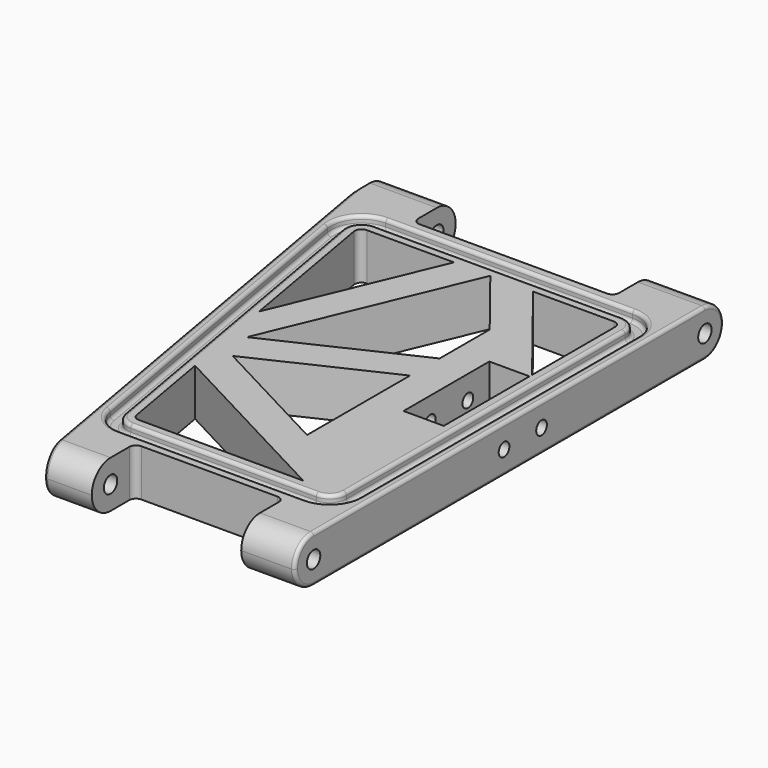
from build123d import *

# Parameters (mm, degrees)
F1_DEPTH  = 3.5
F3_R      = 1.25
F4_DEPTH  = 50.001
F3_R_2    = 1
F5_DEPTH  = 15
F7_DEPTH  = 1.5
F8_R      = 0.5
F9_R      = 0.5
F10_R     = 0.5
F11_R     = 0.5
F13_DEPTH = 1.5
F14_R     = 0.5
F15_R     = 0.5


with BuildPart() as f1:
    # F0 (on Top) → F1 (new body, symmetric)
    with BuildSketch(Plane.XY):
        with BuildLine():
            Line((-29, 45.9712314761), (-39, 45.9712314761))
            Line((-39, 45.9712314761), (-39, 37.9712314761))
            Line((-39, 37.9712314761), (-26.304457389, -34.0287685239))
            Line((-26.304457389, -34.0287685239), (-19.304457389, -34.0287685239))
            Line((-19.304457389, -34.0287685239), (-19.304457389, -27.0287685239))
            ThreePointArc((-19.304457389, -27.0287685239), (-19.0115641702, -26.3216617427), (-18.304457389, -26.0287685239))
            Line((-18.304457389, -26.0287685239), (2, -26.0287685239))
            ThreePointArc((2, -26.0287685239), (2.7071067812, -26.3216617427), (3, -27.0287685239))
            Line((3, -27.0287685239), (3, -34.0287685239))
            Line((3, -34.0287685239), (11, -34.0287685239))
            Line((11, -34.0287685239), (11, 45.9712314761))
            Line((11, 45.9712314761), (1, 45.9712314761))
            Line((1, 45.9712314761), (1, 38.9712314761))
            ThreePointArc((1, 38.9712314761), (0.7071067812, 38.2641246949), (0, 37.9712314761))
            Line((0, 37.9712314761), (-28, 37.9712314761))
            ThreePointArc((-28, 37.9712314761), (-28.7071067812, 38.2641246949), (-29, 38.9712314761))
            Line((-29, 38.9712314761), (-29, 45.9712314761))
        make_face()
        with BuildLine():
            ThreePointArc((5, 36.4712314761), (8.1819805153, 35.1532119914), (9.5, 31.9712314761))
            Line((9.5, 31.9712314761), (9.5, -20.0287685239))
            ThreePointArc((9.5, -20.0287685239), (8.1819805153, -23.2107490392), (5, -24.5287685239))
            Line((5, -24.5287685239), (-22.6804754476, -24.5287685239))
            ThreePointArc((-22.6804754476, -24.5287685239), (-25.5730196912, -23.4759685179), (-27.1121103361, -20.8101853234))
            Line((-27.1121103361, -20.8101853234), (-36.281113333, 31.1898146766))
            ThreePointArc((-36.281113333, 31.1898146766), (-35.2966784385, 34.8637757197), (-31.8494784444, 36.4712314761))
            Line((-31.8494784444, 36.4712314761), (5, 36.4712314761))
        make_face(mode=Mode.SUBTRACT)
        with BuildLine():
            Line((9.5, -20.0287685239), (9.5, 31.9712314761))
            ThreePointArc((9.5, 31.9712314761), (8.1819805153, 35.1532119914), (5, 36.4712314761))
            Line((5, 36.4712314761), (-31.8494784444, 36.4712314761))
            ThreePointArc((-31.8494784444, 36.4712314761), (-35.2966784385, 34.8637757197), (-36.281113333, 31.1898146766))
            Line((-36.281113333, 31.1898146766), (-27.1121103361, -20.8101853234))
            ThreePointArc((-27.1121103361, -20.8101853234), (-25.5730196912, -23.4759685179), (-22.6804754476, -24.5287685239))
            Line((-22.6804754476, -24.5287685239), (5, -24.5287685239))
            ThreePointArc((5, -24.5287685239), (8.1819805153, -23.2107490392), (9.5, -20.0287685239))
        make_face()
        with BuildLine():
            ThreePointArc((5, 34.4712314761), (6.767766953, 33.7389984291), (7.5, 31.9712314761))
            Line((7.5, 31.9712314761), (7.5, -20.0287685239))
            ThreePointArc((7.5, -20.0287685239), (6.767766953, -21.7965354769), (5, -22.5287685239))
            Line((5, -22.5287685239), (-22.6804754476, -22.5287685239))
            ThreePointArc((-22.6804754476, -22.5287685239), (-24.2874444718, -21.9438796317), (-25.1424948301, -20.4628889681))
            Line((-25.1424948301, -20.4628889681), (-34.311497827, 31.5371110319))
            ThreePointArc((-34.311497827, 31.5371110319), (-33.7645895522, 33.5782005003), (-31.8494784444, 34.4712314761))
            Line((-31.8494784444, 34.4712314761), (5, 34.4712314761))
        make_face(mode=Mode.SUBTRACT)
        with BuildLine():
            Line((7.5, -20.0287685239), (7.5, 31.9712314761))
            ThreePointArc((7.5, 31.9712314761), (6.767766953, 33.7389984291), (5, 34.4712314761))
            Line((5, 34.4712314761), (-31.8494784444, 34.4712314761))
            ThreePointArc((-31.8494784444, 34.4712314761), (-33.7645895522, 33.5782005003), (-34.311497827, 31.5371110319))
            Line((-34.311497827, 31.5371110319), (-25.1424948301, -20.4628889681))
            ThreePointArc((-25.1424948301, -20.4628889681), (-24.2874444718, -21.9438796317), (-22.6804754476, -22.5287685239))
            Line((-22.6804754476, -22.5287685239), (5, -22.5287685239))
            ThreePointArc((5, -22.5287685239), (6.767766953, -21.7965354769), (7.5, -20.0287685239))
        make_face()
        with BuildLine():
            Line((6, -17.5660868453), (6, -20.0287685239))
            ThreePointArc((6, -20.0287685239), (5.7071067812, -20.7358753051), (5, -21.0287685239))
            Line((5, -21.0287685239), (1.851729083, -21.0287685239))
            Line((1.851729083, -21.0287685239), (-22.6804754476, -21.0287685239))
            ThreePointArc((-22.6804754476, -21.0287685239), (-23.3232630573, -20.794812967), (-23.6652832006, -20.2024167016))
            Line((-23.6652832006, -20.2024167016), (-26.1277423997, -6.2371166142))
            Line((-26.1277423997, -6.2371166142), (-27.2275143406, 0))
            Line((-27.2275143406, 0), (-28.8339674103, 9.1106480882))
            Line((-28.8339674103, 9.1106480882), (-32.8342861974, 31.7975832984))
            ThreePointArc((-32.8342861974, 31.7975832984), (-32.6155228876, 32.6140190858), (-31.8494784444, 32.9712314761))
            Line((-31.8494784444, 32.9712314761), (-18.8451907723, 32.9712314761))
            Line((-18.8451907723, 32.9712314761), (-13.4247392222, 32.9712314761))
            Line((-13.4247392222, 32.9712314761), (-7.0495389221, 32.9712314761))
            Line((-7.0495389221, 32.9712314761), (5, 32.9712314761))
            ThreePointArc((5, 32.9712314761), (5.7071067812, 32.6783382573), (6, 31.9712314761))
            Line((6, 31.9712314761), (6, 16.4743191684))
            Line((6, 16.4743191684), (6, 16))
            Line((6, 16), (6, 0))
            Line((6, 0), (6, -17.5660868453))
        make_face(mode=Mode.SUBTRACT)
        with BuildLine():
            ThreePointArc((5, -21.0287685239), (5.7071067812, -20.7358753051), (6, -20.0287685239))
            Line((6, -20.0287685239), (6, -17.5660868453))
            Line((6, -17.5660868453), (-5, -11.7508172071))
            Line((-5, -11.7508172071), (-24.2358700371, -1.5815652988))
            Line((-24.2358700371, -1.5815652988), (-27.2275143406, 0))
            Line((-27.2275143406, 0), (-26.1277423997, -6.2371166142))
            Line((-26.1277423997, -6.2371166142), (1.851729083, -21.0287685239))
            Line((1.851729083, -21.0287685239), (5, -21.0287685239))
        make_face()
        Polygon((-27.2275143406, 0), (-24.2358700371, -1.5815652988), (-5, 7.4545675071), (-5, 12.9787622658), (-25.9053092883, 3.1584031808), align=None)
        Polygon((-28.8339674103, 9.1106480882), (-27.2275143406, 0), (-25.9053092883, 3.1584031808), (-13.4247392222, 32.9712314761), (-18.8451907723, 32.9712314761), align=None)
        Polygon((-5, -11.7508172071), (6, -17.5660868453), (6, 0), (0, 0), (0, 16), (-5, 22.3208793836), (-5, 12.9787622658), (-5, 7.4545675071), align=None)
        Polygon((0, 16), (6, 16), (6, 16.4743191684), (-7.0495389221, 32.9712314761), (-13.4247392222, 32.9712314761), (-5, 22.3208793836), align=None)
    extrude(amount=F1_DEPTH, both=True)

    # F3 (on face) → F4 (cut, through all)
    with BuildSketch(Plane.YZ.offset(11)):
        with BuildLine():
            ThreePointArc((-34.0287685239, 0), (-33.0036422525, 2.4748737397), (-30.5287685081, 3.5))
            Line((-30.5287685081, 3.5), (-34.0287685239, 3.5))
            Line((-34.0287685239, 3.5), (-34.0287685239, 0))
        make_face()
        with BuildLine():
            Line((-34.0287685239, -3.5), (-30.5287685239, -3.5))
            ThreePointArc((-30.5287685239, -3.5), (-33.0036422581, -2.4748737342), (-34.0287685239, 0))
            Line((-34.0287685239, 0), (-34.0287685239, -3.5))
        make_face()
        with BuildLine():
            ThreePointArc((42.4712314761, 3.5), (44.9461052103, 2.4748737342), (45.9712314761, 0))
            Line((45.9712314761, 0), (45.9712314761, 3.5))
            Line((45.9712314761, 3.5), (42.4712314761, 3.5))
        make_face()
        with BuildLine():
            Line((45.9712314761, -3.5), (45.9712314761, 0))
            ThreePointArc((45.9712314761, 0), (44.9461052012, -2.4748737432), (42.4712314506, -3.5))
            Line((42.4712314506, -3.5), (45.9712314761, -3.5))
        make_face()
        with Locations((42.4712314761, 0)):
            Circle(F3_R)
        with Locations((-30.5287685239, 0)):
            Circle(F3_R)
    extrude(amount=-F4_DEPTH, mode=Mode.SUBTRACT)

    # F3 (on face) → F5 (cut)
    with BuildSketch(Plane.YZ.offset(11)):
        with Locations((5, 0)):
            Circle(F3_R_2)
        with Locations((12, 0)):
            Circle(F3_R_2)
    extrude(amount=-F5_DEPTH, mode=Mode.SUBTRACT)

    # F6 (on face) → F7 (cut)
    with BuildSketch(Plane.XY.offset(3.5)):
        with BuildLine():
            Line((5, 36.4712314761), (-31.8494784444, 36.4712314761))
            ThreePointArc((-31.8494784444, 36.4712314761), (-35.2966784385, 34.8637757197), (-36.281113333, 31.1898146766))
            Line((-36.281113333, 31.1898146766), (-27.1121103361, -20.8101853234))
            ThreePointArc((-27.1121103361, -20.8101853234), (-25.5730196912, -23.4759685179), (-22.6804754476, -24.5287685239))
            Line((-22.6804754476, -24.5287685239), (5, -24.5287685239))
            ThreePointArc((5, -24.5287685239), (8.1819805153, -23.2107490392), (9.5, -20.0287685239))
            Line((9.5, -20.0287685239), (9.5, 31.9712314761))
            ThreePointArc((9.5, 31.9712314761), (8.1819805153, 35.1532119914), (5, 36.4712314761))
        make_face()
        with BuildLine():
            Line((-31.8494784444, 34.4712314761), (5, 34.4712314761))
            ThreePointArc((5, 34.4712314761), (6.767766953, 33.7389984291), (7.5, 31.9712314761))
            Line((7.5, 31.9712314761), (7.5, -20.0287685239))
            ThreePointArc((7.5, -20.0287685239), (6.767766953, -21.7965354769), (5, -22.5287685239))
            Line((5, -22.5287685239), (-22.6804754476, -22.5287685239))
            ThreePointArc((-22.6804754476, -22.5287685239), (-24.2874444718, -21.9438796317), (-25.1424948301, -20.4628889681))
            Line((-25.1424948301, -20.4628889681), (-34.311497827, 31.5371110319))
            ThreePointArc((-34.311497827, 31.5371110319), (-33.7645895522, 33.5782005003), (-31.8494784444, 34.4712314761))
        make_face(mode=Mode.SUBTRACT)
    extrude(amount=-F7_DEPTH, mode=Mode.SUBTRACT)

    # F8
    f8_edges = [f1.edges().sort_by_distance(p)[0] for p in [
        (-31.696612, 5.189815, 3.5),
        (-29.726996, 5.537111, 3.5),
    ]]
    fillet(f8_edges, radius=F8_R)

    # F9
    f9_edges = [f1.edges().sort_by_distance(p)[0] for p in [
        (8.181981, 35.153212, 2),
        (-13.424739, 36.471231, 2),
        (-35.296678, 34.863776, 2),
        (-31.696612, 5.189815, 2),
        (-25.57302, -23.475969, 2),
        (-8.840238, -24.528769, 2),
        (8.181981, -23.210749, 2),
        (9.5, 5.971231, 2),
        (-13.424739, 34.471231, 2),
        (6.767767, 33.738998, 2),
        (7.5, 5.971231, 2),
        (6.767767, -21.796535, 2),
        (-8.840238, -22.528769, 2),
        (-24.287444, -21.94388, 2),
        (-29.726996, 5.537111, 2),
        (-33.76459, 33.578201, 2),
    ]]
    fillet(f9_edges, radius=F9_R)

    # F10
    f10_edges = [f1.edges().sort_by_distance(p)[0] for p in [
        (-32.960801, 3.721231, 3.5),
    ]]
    fillet(f10_edges, radius=F10_R)

    # F11
    f11_edges = [f1.edges().sort_by_distance(p)[0] for p in [
        (11, 5.971231, 3.5),
        (11, -34.028769, 0),
        (11, 5.971231, -3.5),
        (11, 45.971231, 0),
    ]]
    fillet(f11_edges, radius=F11_R)

    # F12 (on face) → F13 (cut)
    with BuildSketch(Plane(origin=(0, 0, -3.5), x_dir=(1, 0, 0), z_dir=(0, 0, -1))):
        with BuildLine():
            ThreePointArc((-36.281113333, -31.1898146766), (-35.2966784385, -34.8637757197), (-31.8494784444, -36.4712314761))
            Line((-31.8494784444, -36.4712314761), (5, -36.4712314761))
            ThreePointArc((5, -36.4712314761), (8.1819805153, -35.1532119914), (9.5, -31.9712314761))
            Line((9.5, -31.9712314761), (9.5, 20.0287685239))
            ThreePointArc((9.5, 20.0287685239), (8.1819805153, 23.2107490392), (5, 24.5287685239))
            Line((5, 24.5287685239), (-22.6804754476, 24.5287685239))
            ThreePointArc((-22.6804754476, 24.5287685239), (-25.5730196912, 23.4759685179), (-27.1121103361, 20.8101853234))
            Line((-27.1121103361, 20.8101853234), (-36.281113333, -31.1898146766))
        make_face()
        with BuildLine():
            ThreePointArc((7.5, -31.9712314761), (6.767766953, -33.7389984291), (5, -34.4712314761))
            Line((5, -34.4712314761), (-31.8494784444, -34.4712314761))
            ThreePointArc((-31.8494784444, -34.4712314761), (-33.7645895522, -33.5782005003), (-34.311497827, -31.5371110319))
            Line((-34.311497827, -31.5371110319), (-25.1424948301, 20.4628889681))
            ThreePointArc((-25.1424948301, 20.4628889681), (-24.2874444718, 21.9438796317), (-22.6804754476, 22.5287685239))
            Line((-22.6804754476, 22.5287685239), (5, 22.5287685239))
            ThreePointArc((5, 22.5287685239), (6.767766953, 21.7965354769), (7.5, 20.0287685239))
            Line((7.5, 20.0287685239), (7.5, -31.9712314761))
        make_face(mode=Mode.SUBTRACT)
    extrude(amount=-F13_DEPTH, mode=Mode.SUBTRACT)

    # F14
    f14_edges = [f1.edges().sort_by_distance(p)[0] for p in [
        (-31.696612, 5.189815, -3.5),
        (-29.726996, 5.537111, -3.5),
    ]]
    fillet(f14_edges, radius=F14_R)

    # F15
    f15_edges = [f1.edges().sort_by_distance(p)[0] for p in [
        (-35.296678, 34.863776, -2),
        (-13.424739, 36.471231, -2),
        (8.181981, 35.153212, -2),
        (9.5, 5.971231, -2),
        (8.181981, -23.210749, -2),
        (-8.840238, -24.528769, -2),
        (-25.57302, -23.475969, -2),
        (-31.696612, 5.189815, -2),
        (6.767767, -21.796535, -2),
        (7.5, 5.971231, -2),
        (6.767767, 33.738998, -2),
        (-13.424739, 34.471231, -2),
        (-33.76459, 33.578201, -2),
        (-29.726996, 5.537111, -2),
        (-24.287444, -21.94388, -2),
        (-8.840238, -22.528769, -2),
    ]]
    fillet(f15_edges, radius=F15_R)


solid = f1.part
